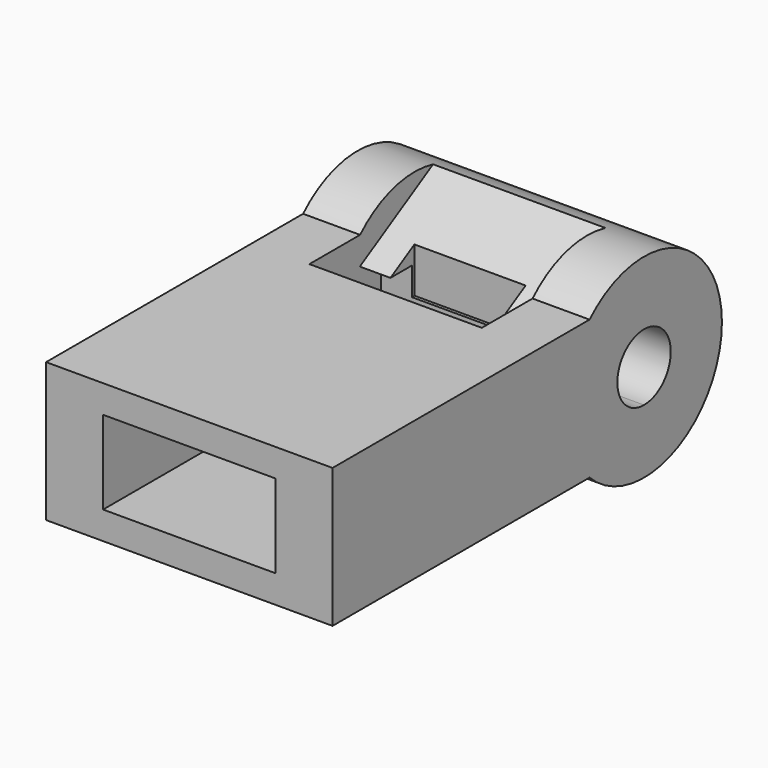
from build123d import *
from build123d import SkipClean  # not in build123d's __all__

# Parameters (mm, degrees)
F0_W          = 10.3
F0_H          = 5
F1_DEPTH      = 10
F3_DEPTH      = 10.3
F4_DEPTH      = 11
F5_W          = 4
F5_H          = 2
F6_DEPTH      = 2
F6_DEPTH_BACK = 5
F7_W          = 6.2
F7_H          = 3
F8_DEPTH      = 8.5
F10_W         = 6.2
F10_H         = 2
F11_DEPTH     = 25
F7_W_2        = 10.3
F7_H_2        = 5
F12_DEPTH     = 4


with BuildPart() as f1:
    # F0 (on Front) → F1 (new body)
    with BuildSketch(Plane.XZ):
        Rectangle(F0_W, F0_H)
    extrude(amount=F1_DEPTH)

    # F2 (on face) → F3 (join)
    with BuildSketch(Plane(origin=(-5.15, 0, 0), x_dir=(0, -1, 0), z_dir=(-1, 0, 0))):
        with BuildLine():
            ThreePointArc((0, -1.2), (-1.2, 0), (0, 1.2))
            Line((0, 1.2), (0, 2.5))
            Line((0, 2.5), (2.4494897428, 2.5))
            ThreePointArc((2.4494897428, 2.5), (-3.5, 0), (2.4494897428, -2.5))
            Line((2.4494897428, -2.5), (0, -2.5))
            Line((0, -2.5), (0, -1.2))
        make_face()
    extrude(amount=-F3_DEPTH)

    # F2 (on face) → F4 (cut)
    with BuildSketch(Plane(origin=(-5.15, 0, 0), x_dir=(0, -1, 0), z_dir=(-1, 0, 0))):
        with BuildLine():
            ThreePointArc((0, -1.2), (0.8485281374, -0.8485281374), (1.2, 0))
            ThreePointArc((1.2, 0), (0.8485281374, 0.8485281374), (0, 1.2))
            Line((0, 1.2), (0, -1.2))
        make_face()
    with SkipClean():  # cleaning this boolean's faces spoils the solid; the shape is the same uncleaned
        extrude(amount=-F4_DEPTH, mode=Mode.SUBTRACT)

    # F5 (on face) → F6 (cut, two sides)
    with BuildSketch(Plane.XY.offset(2.5)) as f6_sk:
        with Locations((0, -2.3844429548)):
            Rectangle(F5_W, F5_H)
    extrude(amount=-F6_DEPTH, mode=Mode.SUBTRACT)
    extrude(f6_sk.sketch, amount=F6_DEPTH_BACK, mode=Mode.SUBTRACT)

    # F7 (on face) → F8 (cut)
    with BuildSketch(Plane.XZ.offset(10)):
        Rectangle(F7_W, F7_H)
    extrude(amount=-F8_DEPTH, mode=Mode.SUBTRACT)

    # F10 (on face) → F11 (cut)
    with BuildSketch(Plane(origin=(0, -6.4174682453, -3.7051270189), x_dir=(1, 0, 0), z_dir=(0, -0.8660254038, -0.5))):
        with Locations((0, 3.5294059198)):
            Rectangle(F10_W, F10_H)
    extrude(amount=-F11_DEPTH, mode=Mode.SUBTRACT)

    # F7 (on face) → F12 (join)
    with BuildSketch(Plane.XZ.offset(10)):
        Rectangle(F7_W_2, F7_H_2)
        Rectangle(F7_W, F7_H, mode=Mode.SUBTRACT)
    extrude(amount=F12_DEPTH)


solid = f1.part
